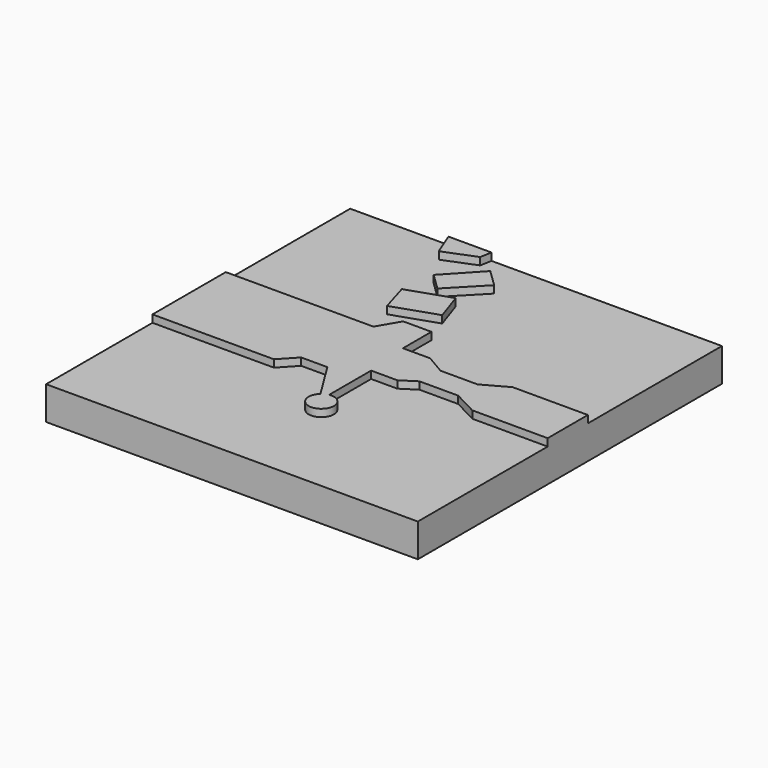
from build123d import *

# Parameters (mm, degrees)
F0_W      = 100.5620509386
F0_H      = 102.8282381594
F1_DEPTH  = 9
F2_R      = 3.4110604721
F3_DEPTH  = 2
F9_DEPTH  = 2
F17_DEPTH = 2
F19_DEPTH = 2
F21_DEPTH = 2


# Not quite as in the source:
# - the program builds the solid bodies; features that only make, move or delete a surface that nothing else refers to are left out


with BuildPart() as f1:
    # F0 (on Top) → F1 (new body)
    with BuildSketch(Plane.XY):
        with Locations((2.2661872208, -9.3480218202)):
            Rectangle(F0_W, F0_H)
    extrude(amount=F1_DEPTH)

    # F2 (on face) → F3 (join)
    with BuildSketch(Plane.XY.offset(9)):
        with Locations((4.6740118414, -33.5678942502)):
            Circle(F2_R)
    extrude(amount=F3_DEPTH)

    # F8 (on face) → F9 (join)
    with BuildSketch(Plane.XY.offset(9)):
        with BuildLine():
            Line((-4.1074641049, -20.5373205245), (2.40785712, -31.0184087486))
            ThreePointArc((2.40785712, -31.0184087486), (3.2003162928, -30.4916050937), (4.1074650362, -30.2042120027))
            Line((4.1074650362, -30.2042120027), (4.1074650362, -16.0049479455))
            Line((4.1074650362, -16.0049479455), (11.1892977729, -16.0049479455))
            Line((11.1892977729, -16.0049479455), (15.155127272, -13.4554868564))
            Line((15.155127272, -13.4554868564), (25.63624084, -13.4554868564))
            Line((25.63624084, -13.4554868564), (32.1515314281, -16.8547667563))
            Line((32.1515314281, -16.8547667563), (52.5472126901, -16.8547667563))
            Line((52.5472126901, -16.8547667563), (52.5472126901, -3.2576438971))
            Line((52.5472126901, -3.2576438971), (32.1515314281, -3.2576438971))
            Line((32.1515314281, -3.2576438971), (25.63624084, -6.8936358156))
            Line((25.63624084, -6.8936358156), (15.5831124042, -6.8936358156))
            Line((15.5831124042, -6.8936358156), (10.3394780308, -3.8241909351))
            Line((10.3394780308, -3.8241909351), (2.9743718915, -3.8241909351))
            Line((2.9743718915, -3.8241909351), (2.9743718915, 5.8071040548))
            Line((2.9743718915, 5.8071040548), (-4.6740109101, 5.8071040548))
            Line((-4.6740109101, 5.8071040548), (-8.0732917413, 0))
            Line((-8.0732917413, 0), (-48.0148382485, 0))
            Line((-48.0148382485, 0), (-48.0148382485, -24.7864220291))
            Line((-48.0148382485, -24.7864220291), (-15.1551263407, -24.7864220291))
            Line((-15.1551263407, -24.7864220291), (-11.1892987043, -20.5373205245))
            Line((-11.1892987043, -20.5373205245), (-4.1074641049, -20.5373205245))
        make_face()
    extrude(amount=F9_DEPTH)

    # F16 (on face) → F17 (join)
    with BuildSketch(Plane.XY.offset(9)):
        Polygon((-14.1233374194, 17.1550600206), (-11.7558455095, 9.2063853517), (0, 13.1722129881), (-2.6493984959, 21.0257866344), align=None)
    extrude(amount=F17_DEPTH)

    # F18 (on face) → F19 (join)
    with BuildSketch(Plane.XY.offset(9)):
        Polygon((0, 30.7351611555), (-4.6740109101, 35.2675393224), (-12.9274129612, 26.4375342768), (-8.4126724433, 22.0596002612), align=None)
    extrude(amount=F19_DEPTH)

    # F20 (on face) → F21 (join)
    with BuildSketch(Plane.XY.offset(9)):
        Polygon((-18.8376810402, 35.5508103967), (-10.3394789621, 38.9500930905), (-9.7729321569, 42.0660972595), (-21.4437972133, 42.0660972595), align=None)
    extrude(amount=F21_DEPTH)


solid = f1.part
